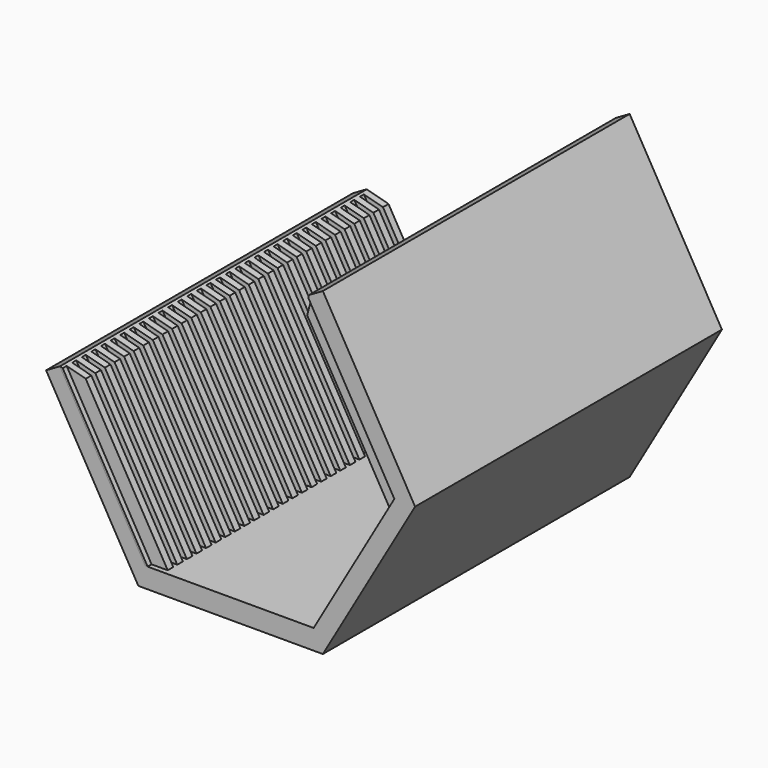
from build123d import *

# Parameters (mm, degrees)
F1_DEPTH     = 48
F3_DEPTH     = 46
F5_DEPTH     = 46
F6_T1_DEPTH  = 22.3234639037
F6_T3_DEPTH  = 22.3234639037
F6_T5_DEPTH  = 22.3234639037
F6_T7_DEPTH  = 22.3234639037
F6_T9_DEPTH  = 22.3234639037
F6_T11_DEPTH = 22.3234639037
F6_T13_DEPTH = 22.3234639037
F6_T15_DEPTH = 22.3234639037
F6_T17_DEPTH = 22.3234639037
F6_T19_DEPTH = 22.3234639037
F6_T21_DEPTH = 22.3234639037
F6_T23_DEPTH = 22.3234639037
F6_T25_DEPTH = 22.3234639037
F6_T27_DEPTH = 22.3234639037
F6_T29_DEPTH = 22.3234639037
F6_T31_DEPTH = 22.3234639037
F6_T33_DEPTH = 22.3234639037
F6_T35_DEPTH = 22.3234639037
F6_T37_DEPTH = 22.3234639037
F6_T39_DEPTH = 22.3234639037
F6_T41_DEPTH = 22.3234639037
F6_T43_DEPTH = 22.3234639037
F6_T45_DEPTH = 22.3234639037
F6_T47_DEPTH = 22.3234639037
F6_T49_DEPTH = 22.3234639037
F6_T51_DEPTH = 22.3234639037
F6_T53_DEPTH = 22.3234639037
F6_T55_DEPTH = 22.3234639037
F6_T57_DEPTH = 22.3234639037
F6_T59_DEPTH = 22.3234639037
F6_T61_DEPTH = 22.3234639037
F6_T63_DEPTH = 22.3234639037


# Not quite as in the source:
# - a fillet or chamfer that OpenCascade refuses, or shapes differently, is made with other operations: its cross-section is extruded or revolved along the edge and cut away or added
# - ends of sketch curves that miss each other by under 0.0002 mm in the source are joined


with BuildPart() as f1:
    # F0 (on Front) → F1 (new body, symmetric)
    with BuildSketch(Plane.XZ):
        Polygon((23.0940107676, -40), (46.1880215352, 0), (23.0940107676, 40), (19.6299091524, 38), (41.2805442471, 0.5), (20.7846096908, -35), (-21.36195996, -35), (-42.72391992, 2), (-46.1880215352, 0), (-23.0940107676, -40), align=None)
    extrude(amount=F1_DEPTH, both=True)

    # F2 (on face) → F3 (join)
    with BuildSketch(Plane(origin=(-11.5470053838, 0, 20), x_dir=(0.8660254038, 0, 0.5), z_dir=(-0.5, 0, 0.8660254038))):
        Polygon((-32, 46.25), (-32, 48), (-35.5, 48), (-36, 48), (-36, -48), (-35.4984295879, -47.9999990135), (-35.5, -46.75), (-32, -46.75), (-32, -45), (-35.4984295879, -45), (-35.5, -43.75), (-32, -43.75), (-32, -42), (-35.4984295879, -42), (-35.5, -40.75), (-32, -40.75), (-32, -39), (-35.4984295879, -39), (-35.5, -37.75), (-32, -37.75), (-32, -36), (-35.4984295879, -36), (-35.5, -34.75), (-32, -34.75), (-32, -33), (-35.4984295879, -33), (-35.5, -31.75), (-32, -31.75), (-32, -30), (-35.4984295879, -30), (-35.5, -28.75), (-32, -28.75), (-32, -27), (-35.4984295879, -27), (-35.5, -25.75), (-32, -25.75), (-32, -24), (-35.4984295879, -24), (-35.5, -22.75), (-32, -22.75), (-32, -21), (-35.4984295879, -21), (-35.5, -19.75), (-32, -19.75), (-32, -18), (-35.4984295879, -18), (-35.5, -16.75), (-32, -16.75), (-32, -15), (-35.4984295879, -15), (-35.5, -13.75), (-32, -13.75), (-32, -12), (-35.4984295879, -12), (-35.5, -10.75), (-32, -10.75), (-32, -9), (-35.4984295879, -9), (-35.5, -7.75), (-32, -7.75), (-32, -6), (-35.4984295879, -6), (-35.5, -4.75), (-32, -4.75), (-32, -3), (-35.4984295879, -3), (-35.5, -1.75), (-32, -1.75), (-32, 0), (-35.4984295879, 0), (-35.5, 1.25), (-32, 1.25), (-32, 3), (-35.4984295879, 3), (-35.5, 4.25), (-32, 4.25), (-32, 6), (-35.4984295879, 6), (-35.5, 7.25), (-32, 7.25), (-32, 9), (-35.4984295879, 9), (-35.5, 10.25), (-32, 10.25), (-32, 12), (-35.4984295879, 12), (-35.5, 13.25), (-32, 13.25), (-32, 15), (-35.4984295879, 15), (-35.5, 16.25), (-32, 16.25), (-32, 18), (-35.4984295879, 18), (-35.5, 19.25), (-32, 19.25), (-32, 21), (-35.4984295879, 21), (-35.5, 22.25), (-32, 22.25), (-32, 24), (-35.4984295879, 24), (-35.5, 25.25), (-32, 25.25), (-32, 27), (-35.4984295879, 27), (-35.5, 28.25), (-32, 28.25), (-32, 30), (-35.4984295879, 30), (-35.5, 31.25), (-32, 31.25), (-32, 33), (-35.4984295879, 33), (-35.5, 34.25), (-32, 34.25), (-32, 36), (-35.4984295879, 36), (-35.5, 37.25), (-32, 37.25), (-32, 39), (-35.4984295879, 39), (-35.5, 40.25), (-32, 40.25), (-32, 42), (-35.4984295879, 42), (-35.5, 43.25), (-32, 43.25), (-32, 45), (-35.4984295879, 45), (-35.5, 46.25), align=None)
    extrude(amount=-F3_DEPTH)

    # F4 (on face) → F5 (join)
    with BuildSketch(Plane(origin=(-11.5470053838, 0, 20), x_dir=(0.8660254038, 0, 0.5), z_dir=(-0.5, 0, 0.8660254038))):
        Polygon((36, -48), (36, 48), (35.5, 48), (32, 48), (32, 46.25), (35.5, 46.25), (35.5, 45), (32, 45), (32, 43.25), (35.5, 43.25), (35.5, 42), (32, 42), (32, 40.25), (35.5, 40.25), (35.5, 39), (32, 39), (32, 37.25), (35.5, 37.25), (35.5, 36), (32, 36), (32, 34.25), (35.5, 34.25), (35.5, 33), (32, 33), (32, 31.25), (35.5, 31.25), (35.5, 30), (32, 30), (32, 28.25), (35.5, 28.25), (35.5, 27), (32, 27), (32, 25.25), (35.5, 25.25), (35.5, 24), (32, 24), (32, 22.25), (35.5, 22.25), (35.5, 21), (32, 21), (32, 19.25), (35.5, 19.25), (35.5, 18), (32, 18), (32, 16.25), (35.5, 16.25), (35.5, 15), (32, 15), (32, 13.25), (35.5, 13.25), (35.5, 12), (32, 12), (32, 10.25), (35.5, 10.25), (35.5, 9), (32, 9), (32, 7.25), (35.5, 7.25), (35.5, 6), (32, 6), (32, 4.25), (35.5, 4.25), (35.5, 3), (32, 3), (32, 1.25), (35.5, 1.25), (35.5, 0), (32, 0), (32, -1.75), (35.5, -1.75), (35.5, -3), (32, -3), (32, -4.75), (35.5, -4.75), (35.5, -6), (32, -6), (32, -7.75), (35.5, -7.75), (35.5, -9), (32, -9), (32, -10.75), (35.5, -10.75), (35.5, -12), (32, -12), (32, -13.75), (35.5, -13.75), (35.5, -15), (32, -15), (32, -16.75), (35.5, -16.75), (35.5, -18), (32, -18), (32, -19.75), (35.5, -19.75), (35.5, -21), (32, -21), (32, -22.75), (35.5, -22.75), (35.5, -24), (32, -24), (32, -25.75), (35.5, -25.75), (35.5, -27), (32, -27), (32, -28.75), (35.5, -28.75), (35.5, -30), (32, -30), (32, -31.75), (35.5, -31.75), (35.5, -33), (32, -33), (32, -34.75), (35.5, -34.75), (35.5, -36), (32, -36), (32, -37.75), (35.5, -37.75), (35.5, -39), (32, -39), (32, -40.75), (35.5, -40.75), (35.5, -42), (32, -42), (32, -43.75), (35.5, -43.75), (35.5, -45), (32, -45), (32, -46.75), (35.5, -46.75), (35.5, -48), align=None)
    extrude(amount=-F5_DEPTH)

    # F6: chamfer of 4 on 64 edges, made by hand

    # F6_s2 → F6_t1 (cut)
    with BuildSketch(Plane.XZ.offset(-58.2867319519)):
        Polygon((-42.72391992, 2), (-37.2598183049, 0.5358983849), (-39.2598183049, 4), align=None)
        Polygon((19.6299091524, 38), (18.1658075373, 32.5358983849), (16.1658075373, 36), align=None)
    extrude(amount=F6_T1_DEPTH, mode=Mode.SUBTRACT)

    # F6_s4 → F6_t3 (cut)
    with BuildSketch(Plane.XZ.offset(34.7132680481)):
        Polygon((19.6299091524, 38), (18.1658075373, 32.5358983849), (16.1658075373, 36), align=None)
        Polygon((-42.72391992, 2), (-37.2598183049, 0.5358983849), (-39.2598183049, 4), align=None)
    extrude(amount=F6_T3_DEPTH, mode=Mode.SUBTRACT)

    # F6_s6 → F6_t5 (cut)
    with BuildSketch(Plane.XZ.offset(31.7132680481)):
        Polygon((-42.72391992, 2), (-37.2598183049, 0.5358983849), (-39.2598183049, 4), align=None)
        Polygon((19.6299091524, 38), (18.1658075373, 32.5358983849), (16.1658075373, 36), align=None)
    extrude(amount=F6_T5_DEPTH, mode=Mode.SUBTRACT)

    # F6_s8 → F6_t7 (cut)
    with BuildSketch(Plane.XZ.offset(28.7132680481)):
        Polygon((-42.72391992, 2), (-37.2598183049, 0.5358983849), (-39.2598183049, 4), align=None)
        Polygon((19.6299091524, 38), (18.1658075373, 32.5358983849), (16.1658075373, 36), align=None)
    extrude(amount=F6_T7_DEPTH, mode=Mode.SUBTRACT)

    # F6_s10 → F6_t9 (cut)
    with BuildSketch(Plane.XZ.offset(25.7132680481)):
        Polygon((-42.72391992, 2), (-37.2598183049, 0.5358983849), (-39.2598183049, 4), align=None)
        Polygon((19.6299091524, 38), (18.1658075373, 32.5358983849), (16.1658075373, 36), align=None)
    extrude(amount=F6_T9_DEPTH, mode=Mode.SUBTRACT)

    # F6_s12 → F6_t11 (cut)
    with BuildSketch(Plane.XZ.offset(22.7132680481)):
        Polygon((-42.72391992, 2), (-37.2598183049, 0.5358983849), (-39.2598183049, 4), align=None)
        Polygon((19.6299091524, 38), (18.1658075373, 32.5358983849), (16.1658075373, 36), align=None)
    extrude(amount=F6_T11_DEPTH, mode=Mode.SUBTRACT)

    # F6_s14 → F6_t13 (cut)
    with BuildSketch(Plane.XZ.offset(19.7132680481)):
        Polygon((-42.72391992, 2), (-37.2598183049, 0.5358983849), (-39.2598183049, 4), align=None)
        Polygon((19.6299091524, 38), (18.1658075373, 32.5358983849), (16.1658075373, 36), align=None)
    extrude(amount=F6_T13_DEPTH, mode=Mode.SUBTRACT)

    # F6_s16 → F6_t15 (cut)
    with BuildSketch(Plane.XZ.offset(16.7132680481)):
        Polygon((-42.72391992, 2), (-37.2598183049, 0.5358983849), (-39.2598183049, 4), align=None)
        Polygon((19.6299091524, 38), (18.1658075373, 32.5358983849), (16.1658075373, 36), align=None)
    extrude(amount=F6_T15_DEPTH, mode=Mode.SUBTRACT)

    # F6_s18 → F6_t17 (cut)
    with BuildSketch(Plane.XZ.offset(13.7132680481)):
        Polygon((-42.72391992, 2), (-37.2598183049, 0.5358983849), (-39.2598183049, 4), align=None)
        Polygon((19.6299091524, 38), (18.1658075373, 32.5358983849), (16.1658075373, 36), align=None)
    extrude(amount=F6_T17_DEPTH, mode=Mode.SUBTRACT)

    # F6_s20 → F6_t19 (cut)
    with BuildSketch(Plane.XZ.offset(10.7132680481)):
        Polygon((-42.72391992, 2), (-37.2598183049, 0.5358983849), (-39.2598183049, 4), align=None)
        Polygon((19.6299091524, 38), (18.1658075373, 32.5358983849), (16.1658075373, 36), align=None)
    extrude(amount=F6_T19_DEPTH, mode=Mode.SUBTRACT)

    # F6_s22 → F6_t21 (cut)
    with BuildSketch(Plane.XZ.offset(7.7132680481)):
        Polygon((-42.72391992, 2), (-37.2598183049, 0.5358983849), (-39.2598183049, 4), align=None)
        Polygon((19.6299091524, 38), (18.1658075373, 32.5358983849), (16.1658075373, 36), align=None)
    extrude(amount=F6_T21_DEPTH, mode=Mode.SUBTRACT)

    # F6_s24 → F6_t23 (cut)
    with BuildSketch(Plane.XZ.offset(4.7132680481)):
        Polygon((-42.72391992, 2), (-37.2598183049, 0.5358983849), (-39.2598183049, 4), align=None)
        Polygon((19.6299091524, 38), (18.1658075373, 32.5358983849), (16.1658075373, 36), align=None)
    extrude(amount=F6_T23_DEPTH, mode=Mode.SUBTRACT)

    # F6_s26 → F6_t25 (cut)
    with BuildSketch(Plane.XZ.offset(1.7132680481)):
        Polygon((-42.72391992, 2), (-37.2598183049, 0.5358983849), (-39.2598183049, 4), align=None)
        Polygon((19.6299091524, 38), (18.1658075373, 32.5358983849), (16.1658075373, 36), align=None)
    extrude(amount=F6_T25_DEPTH, mode=Mode.SUBTRACT)

    # F6_s28 → F6_t27 (cut)
    with BuildSketch(Plane.XZ.offset(-1.2867319519)):
        Polygon((-42.72391992, 2), (-37.2598183049, 0.5358983849), (-39.2598183049, 4), align=None)
        Polygon((19.6299091524, 38), (18.1658075373, 32.5358983849), (16.1658075373, 36), align=None)
    extrude(amount=F6_T27_DEPTH, mode=Mode.SUBTRACT)

    # F6_s30 → F6_t29 (cut)
    with BuildSketch(Plane.XZ.offset(-4.2867319519)):
        Polygon((-42.72391992, 2), (-37.2598183049, 0.5358983849), (-39.2598183049, 4), align=None)
        Polygon((19.6299091524, 38), (18.1658075373, 32.5358983849), (16.1658075373, 36), align=None)
    extrude(amount=F6_T29_DEPTH, mode=Mode.SUBTRACT)

    # F6_s32 → F6_t31 (cut)
    with BuildSketch(Plane.XZ.offset(-7.2867319519)):
        Polygon((-42.72391992, 2), (-37.2598183049, 0.5358983849), (-39.2598183049, 4), align=None)
        Polygon((19.6299091524, 38), (18.1658075373, 32.5358983849), (16.1658075373, 36), align=None)
    extrude(amount=F6_T31_DEPTH, mode=Mode.SUBTRACT)

    # F6_s34 → F6_t33 (cut)
    with BuildSketch(Plane.XZ.offset(-10.2867319519)):
        Polygon((-42.72391992, 2), (-37.2598183049, 0.5358983849), (-39.2598183049, 4), align=None)
        Polygon((19.6299091524, 38), (18.1658075373, 32.5358983849), (16.1658075373, 36), align=None)
    extrude(amount=F6_T33_DEPTH, mode=Mode.SUBTRACT)

    # F6_s36 → F6_t35 (cut)
    with BuildSketch(Plane.XZ.offset(-13.2867319519)):
        Polygon((-42.72391992, 2), (-37.2598183049, 0.5358983849), (-39.2598183049, 4), align=None)
        Polygon((19.6299091524, 38), (18.1658075373, 32.5358983849), (16.1658075373, 36), align=None)
    extrude(amount=F6_T35_DEPTH, mode=Mode.SUBTRACT)

    # F6_s38 → F6_t37 (cut)
    with BuildSketch(Plane.XZ.offset(-16.2867319519)):
        Polygon((-42.72391992, 2), (-37.2598183049, 0.5358983849), (-39.2598183049, 4), align=None)
        Polygon((19.6299091524, 38), (18.1658075373, 32.5358983849), (16.1658075373, 36), align=None)
    extrude(amount=F6_T37_DEPTH, mode=Mode.SUBTRACT)

    # F6_s40 → F6_t39 (cut)
    with BuildSketch(Plane.XZ.offset(-19.2867319519)):
        Polygon((-42.72391992, 2), (-37.2598183049, 0.5358983849), (-39.2598183049, 4), align=None)
        Polygon((19.6299091524, 38), (18.1658075373, 32.5358983849), (16.1658075373, 36), align=None)
    extrude(amount=F6_T39_DEPTH, mode=Mode.SUBTRACT)

    # F6_s42 → F6_t41 (cut)
    with BuildSketch(Plane.XZ.offset(-22.2867319519)):
        Polygon((-42.72391992, 2), (-37.2598183049, 0.5358983849), (-39.2598183049, 4), align=None)
        Polygon((19.6299091524, 38), (18.1658075373, 32.5358983849), (16.1658075373, 36), align=None)
    extrude(amount=F6_T41_DEPTH, mode=Mode.SUBTRACT)

    # F6_s44 → F6_t43 (cut)
    with BuildSketch(Plane.XZ.offset(-25.2867319519)):
        Polygon((-42.72391992, 2), (-37.2598183049, 0.5358983849), (-39.2598183049, 4), align=None)
        Polygon((19.6299091524, 38), (18.1658075373, 32.5358983849), (16.1658075373, 36), align=None)
    extrude(amount=F6_T43_DEPTH, mode=Mode.SUBTRACT)

    # F6_s46 → F6_t45 (cut)
    with BuildSketch(Plane.XZ.offset(-28.2867319519)):
        Polygon((-42.72391992, 2), (-37.2598183049, 0.5358983849), (-39.2598183049, 4), align=None)
        Polygon((19.6299091524, 38), (18.1658075373, 32.5358983849), (16.1658075373, 36), align=None)
    extrude(amount=F6_T45_DEPTH, mode=Mode.SUBTRACT)

    # F6_s48 → F6_t47 (cut)
    with BuildSketch(Plane.XZ.offset(-31.2867319519)):
        Polygon((-42.72391992, 2), (-37.2598183049, 0.5358983849), (-39.2598183049, 4), align=None)
        Polygon((19.6299091524, 38), (18.1658075373, 32.5358983849), (16.1658075373, 36), align=None)
    extrude(amount=F6_T47_DEPTH, mode=Mode.SUBTRACT)

    # F6_s50 → F6_t49 (cut)
    with BuildSketch(Plane.XZ.offset(-34.2867319519)):
        Polygon((-42.72391992, 2), (-37.2598183049, 0.5358983849), (-39.2598183049, 4), align=None)
        Polygon((19.6299091524, 38), (18.1658075373, 32.5358983849), (16.1658075373, 36), align=None)
    extrude(amount=F6_T49_DEPTH, mode=Mode.SUBTRACT)

    # F6_s52 → F6_t51 (cut)
    with BuildSketch(Plane.XZ.offset(-37.2867319519)):
        Polygon((-42.72391992, 2), (-37.2598183049, 0.5358983849), (-39.2598183049, 4), align=None)
        Polygon((19.6299091524, 38), (18.1658075373, 32.5358983849), (16.1658075373, 36), align=None)
    extrude(amount=F6_T51_DEPTH, mode=Mode.SUBTRACT)

    # F6_s54 → F6_t53 (cut)
    with BuildSketch(Plane.XZ.offset(-40.2867319519)):
        Polygon((-42.72391992, 2), (-37.2598183049, 0.5358983849), (-39.2598183049, 4), align=None)
        Polygon((19.6299091524, 38), (18.1658075373, 32.5358983849), (16.1658075373, 36), align=None)
    extrude(amount=F6_T53_DEPTH, mode=Mode.SUBTRACT)

    # F6_s56 → F6_t55 (cut)
    with BuildSketch(Plane.XZ.offset(-43.2867319519)):
        Polygon((-42.72391992, 2), (-37.2598183049, 0.5358983849), (-39.2598183049, 4), align=None)
        Polygon((19.6299091524, 38), (18.1658075373, 32.5358983849), (16.1658075373, 36), align=None)
    extrude(amount=F6_T55_DEPTH, mode=Mode.SUBTRACT)

    # F6_s58 → F6_t57 (cut)
    with BuildSketch(Plane.XZ.offset(-46.2867319519)):
        Polygon((-42.72391992, 2), (-37.2598183049, 0.5358983849), (-39.2598183049, 4), align=None)
        Polygon((19.6299091524, 38), (18.1658075373, 32.5358983849), (16.1658075373, 36), align=None)
    extrude(amount=F6_T57_DEPTH, mode=Mode.SUBTRACT)

    # F6_s60 → F6_t59 (cut)
    with BuildSketch(Plane.XZ.offset(-49.2867319519)):
        Polygon((-42.72391992, 2), (-37.2598183049, 0.5358983849), (-39.2598183049, 4), align=None)
        Polygon((19.6299091524, 38), (18.1658075373, 32.5358983849), (16.1658075373, 36), align=None)
    extrude(amount=F6_T59_DEPTH, mode=Mode.SUBTRACT)

    # F6_s62 → F6_t61 (cut)
    with BuildSketch(Plane.XZ.offset(-52.2867319519)):
        Polygon((-42.72391992, 2), (-37.2598183049, 0.5358983849), (-39.2598183049, 4), align=None)
        Polygon((19.6299091524, 38), (18.1658075373, 32.5358983849), (16.1658075373, 36), align=None)
    extrude(amount=F6_T61_DEPTH, mode=Mode.SUBTRACT)

    # F6_s64 → F6_t63 (cut)
    with BuildSketch(Plane.XZ.offset(-55.2867319519)):
        Polygon((-42.72391992, 2), (-37.2598183049, 0.5358983849), (-39.2598183049, 4), align=None)
        Polygon((19.6299091524, 38), (18.1658075373, 32.5358983849), (16.1658075373, 36), align=None)
    extrude(amount=F6_T63_DEPTH, mode=Mode.SUBTRACT)


solid = f1.part
